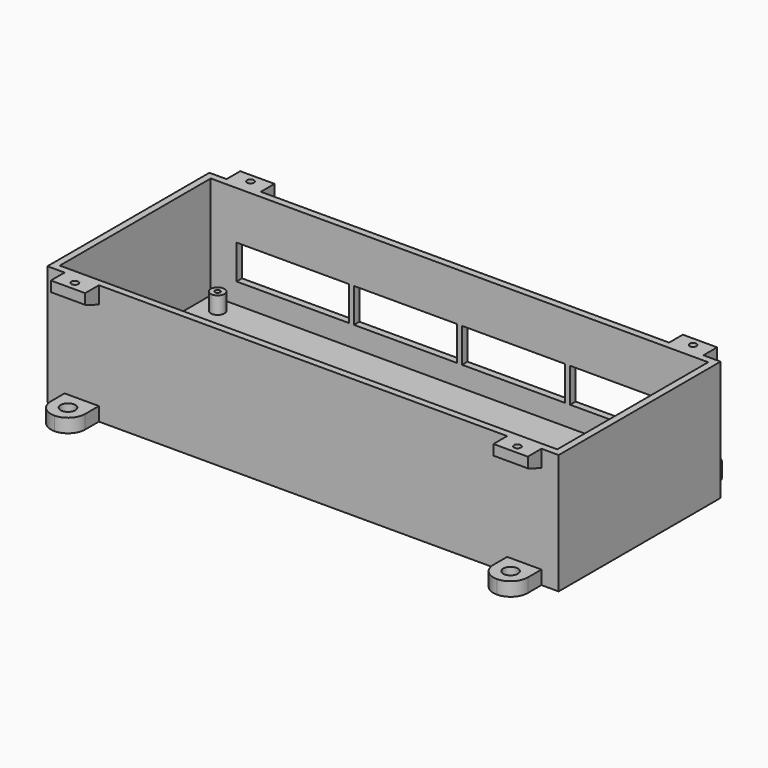
from build123d import *

# Parameters (mm, degrees)
F0_W      = 149
F0_H      = 59
F0_W_2    = 145
F0_H_2    = 55
F1_DEPTH  = 30
F2_W      = 149
F2_H      = 59
F2_W_2    = 145
F2_H_2    = 55
F3_DEPTH  = 5
F4_R      = 2
F4_R_2    = 0.75
F5_DEPTH  = 5
F6_W      = 10
F6_H      = 10
F6_R      = 2.125
F7_DEPTH  = 4
F8_R      = 4.99999
F9_W      = 32.75
F9_H      = 10
F9_W_2    = 30
F10_DEPTH = 2
F11_W     = 10
F11_H     = 5
F12_DEPTH = 5
F14_DEPTH = 144.001
F16_D     = 2
F16_DEPTH = 5
F16_TIP   = 0.600860619


# Not quite as in the source:
# - a fillet or chamfer is up to 0.001 mm smaller than in the source, because OpenCascade refuses the exact size


with BuildPart() as f1:
    # F0 (on Top) → F1 (new body)
    with BuildSketch(Plane.XY):
        Rectangle(F0_W, F0_H)
        Rectangle(F0_W_2, F0_H_2, mode=Mode.SUBTRACT)
    extrude(amount=F1_DEPTH)

    # F2 (on face) → F3 (join)
    with BuildSketch(Plane(origin=(0, 0, 0), x_dir=(1, 0, 0), z_dir=(0, 0, -1))):
        Rectangle(F2_W, F2_H)
        Rectangle(F2_W_2, F2_H_2, mode=Mode.SUBTRACT)
        Rectangle(F2_W_2, F2_H_2)
    extrude(amount=F3_DEPTH)

    # F4 (on face) → F5 (join)
    with BuildSketch(Plane.XY):
        with Locations((-66.5, 22.5)):
            Circle(F4_R)
        with Locations((-66.5, 22.5)):
            Circle(F4_R_2, mode=Mode.SUBTRACT)
        with Locations((-66.5, -22.5)):
            Circle(F4_R)
        with Locations((-66.5, -22.5)):
            Circle(F4_R_2, mode=Mode.SUBTRACT)
        with Locations((66.5, -22.5)):
            Circle(F4_R)
        with Locations((66.5, -22.5)):
            Circle(F4_R_2, mode=Mode.SUBTRACT)
        with Locations((66.5, 22.5)):
            Circle(F4_R)
        with Locations((66.5, 22.5)):
            Circle(F4_R_2, mode=Mode.SUBTRACT)
    extrude(amount=F5_DEPTH)

    # F6 (on face) → F7 (join)
    with BuildSketch(Plane(origin=(0, 0, -5), x_dir=(1, 0, 0), z_dir=(0, 0, -1))):
        with Locations((-64.5, 34.5)):
            Rectangle(F6_W, F6_H)
        with Locations((-64.5, 34.5)):
            Circle(F6_R, mode=Mode.SUBTRACT)
        with Locations((64.5, 34.5)):
            Rectangle(F6_W, F6_H)
        with Locations((64.5, 34.5)):
            Circle(F6_R, mode=Mode.SUBTRACT)
        with Locations((-64.5, -34.5)):
            Rectangle(F6_W, F6_H)
        with Locations((-64.5, -34.5)):
            Circle(F6_R, mode=Mode.SUBTRACT)
        with Locations((64.5, -34.5)):
            Rectangle(F6_W, F6_H)
        with Locations((64.5, -34.5)):
            Circle(F6_R, mode=Mode.SUBTRACT)
    extrude(amount=-F7_DEPTH)

    # F8 (radius 5 in the source; OpenCascade refuses exactly that, so slightly less here)
    f8_edges = [f1.edges().sort_by_distance(p)[0] for p in [
        (-69.5, -39.5, -3),
        (-59.5, -39.5, -3),
        (69.5, -39.5, -3),
        (59.5, -39.5, -3),
        (69.5, 39.5, -3),
        (59.5, 39.5, -3),
        (-59.5, 39.5, -3),
        (-69.5, 39.5, -3),
    ]]
    fillet(f8_edges, radius=F8_R)

    # F9 (on face) → F10 (cut, through all)
    with BuildSketch(Plane(origin=(0, 29.5, 0), x_dir=(-1, 0, 0), z_dir=(0, 1, 0))):
        with Locations((-48.625, 11)):
            Rectangle(F9_W, F9_H)
        with Locations((-15.75, 11)):
            Rectangle(F9_W_2, F9_H)
        with Locations((15.75, 11)):
            Rectangle(F9_W_2, F9_H)
        with Locations((48.625, 11)):
            Rectangle(F9_W, F9_H)
    extrude(amount=-F10_DEPTH, mode=Mode.SUBTRACT)

    # F11 (on face) → F12 (join)
    with BuildSketch(Plane.XY.offset(30)):
        with Locations((64.5, 32)):
            Rectangle(F11_W, F11_H)
        with Locations((-64.5, 32)):
            Rectangle(F11_W, F11_H)
        with Locations((-64.5, -32)):
            Rectangle(F11_W, F11_H)
        with Locations((64.5, -32)):
            Rectangle(F11_W, F11_H)
    extrude(amount=-F12_DEPTH)

    # F13 (on face) → F14 (cut, through all)
    with BuildSketch(Plane(origin=(-69.5, 0, 0), x_dir=(0, -1, 0), z_dir=(-1, 0, 0))):
        Polygon((34.5, 27), (29.5, 25), (34.5, 25), align=None)
        Polygon((-29.5, 25), (-34.5, 27), (-34.5, 25), align=None)
    extrude(amount=-F14_DEPTH, mode=Mode.SUBTRACT)

    # F16
    with Locations(Plane.XY.offset(30)):
        with Locations((64.5, 32), (64.5, -32), (-64.5, -32), (-64.5, 32)):
            Hole(F16_D / 2, depth=F16_DEPTH)
            with Locations((0, 0, -(F16_DEPTH + F16_TIP / 2))):  # 118° drill point
                Cone(0, F16_D / 2, F16_TIP, mode=Mode.SUBTRACT)


solid = f1.part
